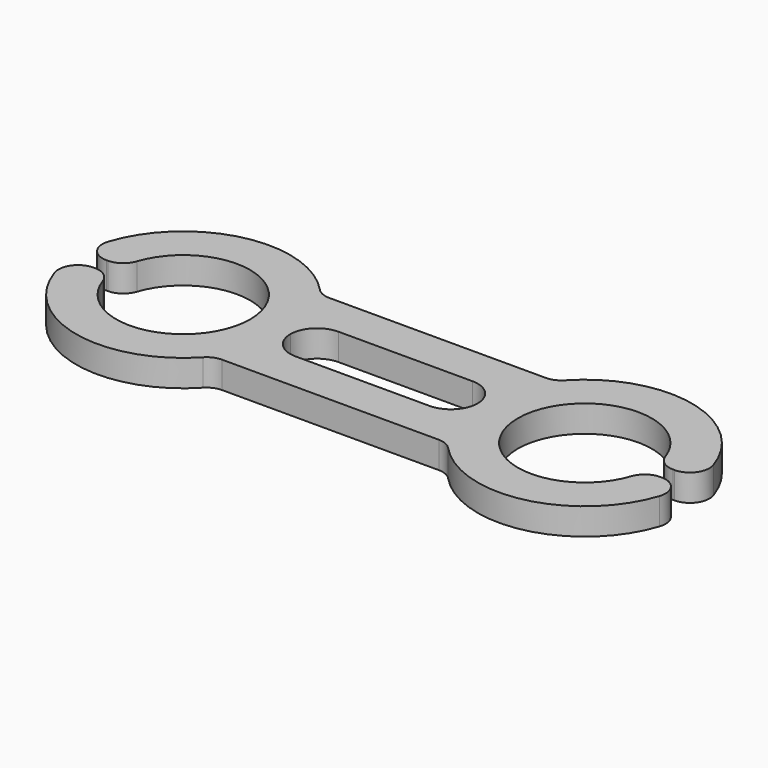
from build123d import *

# Parameters (mm, degrees)
F1_DEPTH = 1.27
F2_R     = 6.35
F3_DEPTH = 25.4
F4_W     = 12.6276115155
F4_H     = 1.524
F5_DEPTH = 25.4
F6_R     = 1.8415
F8_DEPTH = 25.4
F9_R     = 2.53999


# Not quite as in the source:
# - a fillet or chamfer is up to 0.001 mm smaller than in the source, because OpenCascade refuses the exact size


with BuildPart() as f1:
    # F0 (on Top) → F1 (new body, symmetric)
    with BuildSketch(Plane.XY):
        with BuildLine():
            ThreePointArc((-11.118852542, -6.35), (-9.4633932444, -3.3649028089), (-8.89, 0))
            ThreePointArc((-8.89, 0), (-9.4633932444, 3.3649028089), (-11.118852542, 6.35))
            ThreePointArc((-11.118852542, 6.35), (-29.21, 0), (-11.118852542, -6.35))
        make_face()
        with BuildLine():
            ThreePointArc((-11.118852542, 6.35), (-9.4633932444, 3.3649028089), (-8.89, 0))
            ThreePointArc((-8.89, 0), (-9.4633932444, -3.3649028089), (-11.118852542, -6.35))
            Line((-11.118852542, -6.35), (11.118852542, -6.35))
            ThreePointArc((11.118852542, -6.35), (8.89, 0), (11.118852542, 6.35))
            Line((11.118852542, 6.35), (-11.118852542, 6.35))
        make_face()
        with BuildLine():
            ThreePointArc((29.21, 0), (22.4149028089, 9.5866067556), (11.118852542, 6.35))
            ThreePointArc((11.118852542, 6.35), (8.89, 0), (11.118852542, -6.35))
            ThreePointArc((11.118852542, -6.35), (22.4149028089, -9.5866067556), (29.21, 0))
        make_face()
    extrude(amount=F1_DEPTH, both=True)

    # F2 (on face) → F3 (cut)
    with BuildSketch(Plane.XY.offset(1.27)):
        with Locations((-19.05, 0)):
            Circle(F2_R)
        with Locations((19.05, 0)):
            Circle(F2_R)
    extrude(amount=-F3_DEPTH, mode=Mode.SUBTRACT)

    # F4 (on face) → F5 (cut)
    with BuildSketch(Plane.XY.offset(1.27)):
        with Locations((-22.8961942422, 0)):
            Rectangle(F4_W, F4_H)
        with Locations((22.8961942422, 0)):
            Rectangle(F4_W, F4_H)
    extrude(amount=-F5_DEPTH, mode=Mode.SUBTRACT)

    # F6
    f6_edges = [f1.edges().sort_by_distance(p)[0] for p in [
        (-29.181385, 0.762, 0),
        (-25.354114, 0.762, 0),
        (-25.354114, -0.762, 0),
        (-29.181385, -0.762, 0),
        (25.354114, -0.762, 0),
        (25.354114, 0.762, 0),
        (29.181385, 0.762, 0),
        (29.181385, -0.762, 0),
        (-11.118853, -6.35, 0),
        (11.118853, -6.35, 0),
        (11.118853, 6.35, 0),
        (-11.118853, 6.35, 0),
    ]]
    fillet(f6_edges, radius=F6_R)

    # F7 (on face) → F8 (cut)
    with BuildSketch(Plane.XY.offset(1.27)):
        with BuildLine():
            ThreePointArc((-9.2126223006, 2.54), (-8.89, 0), (-9.2126223006, -2.54))
            Line((-9.2126223006, -2.54), (9.2126223006, -2.54))
            ThreePointArc((9.2126223006, -2.54), (8.89, 0), (9.2126223006, 2.54))
            Line((9.2126223006, 2.54), (-9.2126223006, 2.54))
        make_face()
    extrude(amount=-F8_DEPTH, mode=Mode.SUBTRACT)

    # F9 (radius 2.54 in the source; OpenCascade refuses exactly that, so slightly less here)
    f9_edges = [f1.edges().sort_by_distance(p)[0] for p in [
        (-9.212622, -2.54, 0),
        (-9.212622, 2.54, 0),
        (9.212622, 2.54, 0),
        (9.212622, -2.54, 0),
    ]]
    fillet(f9_edges, radius=F9_R)


solid = f1.part
